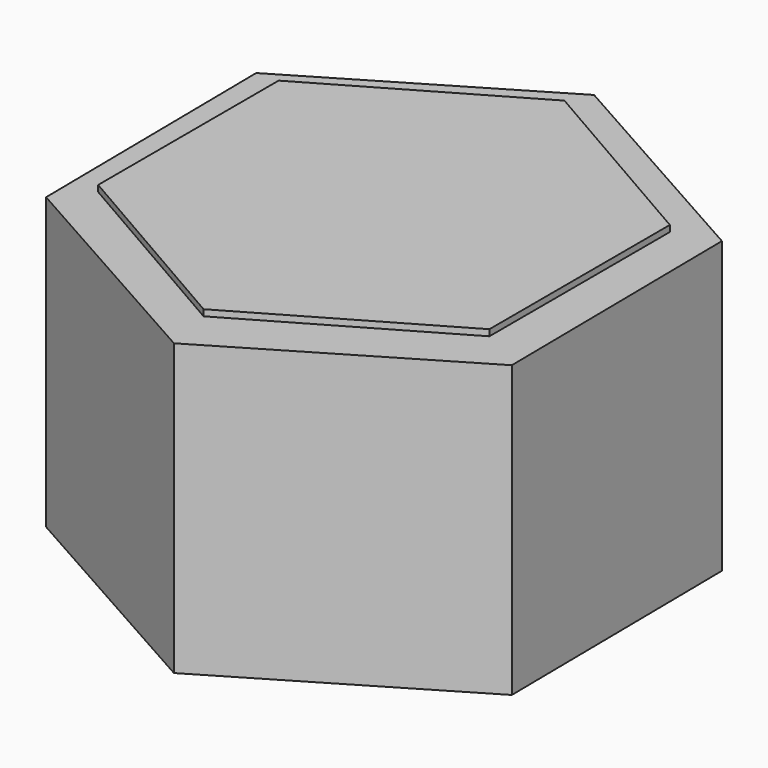
from build123d import *

# Parameters (mm, degrees)
F1_DEPTH  = 56.388
F2_T      = -2.54
F3_W      = 42.9477673024
F3_H      = 39.3949486315
F4_DEPTH  = 25.4
F5_T      = -2.54
F7_DEPTH  = 2.54
F8_R      = 11.4515388828
F9_DEPTH  = 1.27
F11_DEPTH = 1.27


# Not quite as in the source:
# - a shell that OpenCascade refuses in one call is made with other operations: the cavity is built on its own and cut out


with BuildPart() as f1:
    # F0 (on Top) → F1 (new body)
    with BuildSketch(Plane.XY):
        Polygon((46.5280407677, 27.5831491618), (-0.6236875067, 54.0860398741), (-47.1517282744, 26.5028907122), (-46.5280407677, -27.5831491618), (0.6236875067, -54.0860398741), (47.1517282744, -26.5028907122), align=None)
    extrude(amount=F1_DEPTH)

    # F2
    f2_openings = [f1.faces().sort_by_distance(p)[0] for p in [
        (0, 0, 56.388),
    ]]
    offset(amount=F2_T, openings=f2_openings)

    # F3 (on face) → F4 (join)
    with BuildSketch(Plane.XY.offset(2.54)):
        with Locations((-4.2980322614, -2.9984135181)):
            Rectangle(F3_W, F3_H)
    extrude(amount=F4_DEPTH)

    # F5: a shell. OpenCascade refuses it in one call, so the cavity is built on its own and cut out:
    # the body offset inwards by the wall thickness, plus a prism from it out through each open face.
    f5_core = offset(f1.part, amount=F5_T, kind=Kind.INTERSECTION, mode=Mode.PRIVATE)
    f5_exits = [f5_core.faces().sort_by_distance(p)[0] for p in [
        (-4.298032, -2.998414, 25.4),
    ]]
    add(f5_core, mode=Mode.SUBTRACT)
    extrude(f5_exits, amount=-F5_T, mode=Mode.SUBTRACT)

    # F6 (on face) → F7 (join)
    with BuildSketch(Plane.XY.offset(56.388)):
        Polygon((46.5280407677, 27.5831491618), (-0.6236875067, 54.0860398741), (-47.1517282744, 26.5028907122), (-46.5280407677, -27.5831491618), (0.6236875067, -54.0860398741), (47.1517282744, -26.5028907122), align=None)
    extrude(amount=F7_DEPTH)

    # F8 (on face) → F9 (join)
    with BuildSketch(Plane.XY.offset(58.928)):
        Circle(F8_R)
    extrude(amount=F9_DEPTH)

    # F10 (on face) → F11 (join)
    with BuildSketch(Plane.XY.offset(60.198)):
        Polygon((39.6687044392, 22.9401686529), (-0.0324166009, 45.824190106), (-39.7011210401, 22.8840214531), (-39.6687044392, -22.9401686529), (0.0324166009, -45.824190106), (39.7011210401, -22.8840214531), align=None)
    extrude(amount=F11_DEPTH)


solid = f1.part
